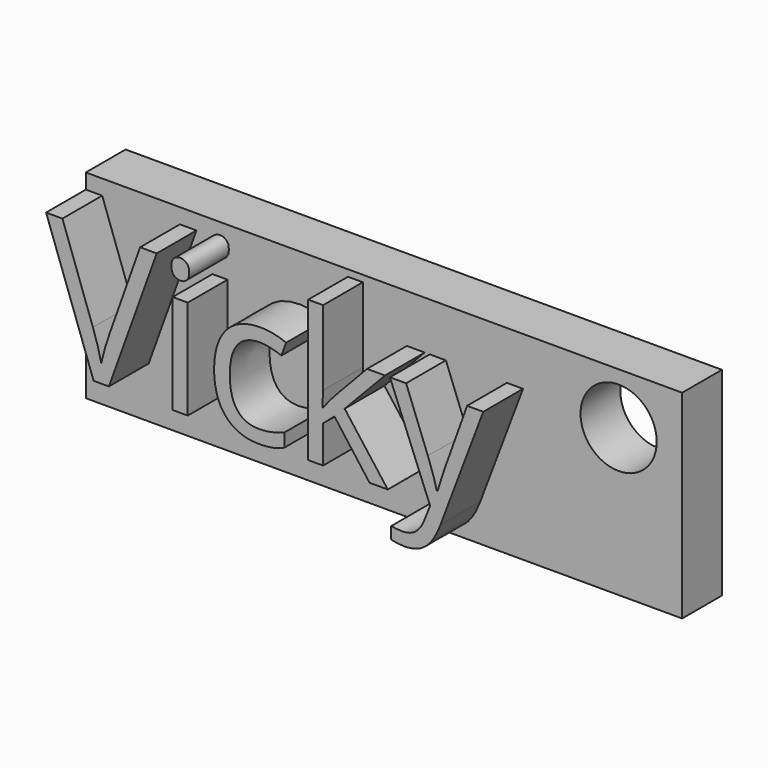
from build123d import *

# Parameters (mm, degrees)
F1_TEXT_SIZE = 23.7509700844
F2_DEPTH     = 12.7
F0_W         = 76.2
F0_H         = 25.4
F3_DEPTH     = 6.35
F4_R         = 4.870183606
F5_DEPTH     = 6.35


# Not quite as in the source:
# - Text() gives the source's letters only with a copy of the font that has no kerning and outlines rounded to 1/6400 em; it was checked with that copy


with BuildPart() as f2:
    # F1 (on face) → F2 (new body)
    with BuildSketch(Plane.XZ):
        with Locations((0, 6.5138929126)):
            Text('Vicky', F1_TEXT_SIZE, font='Open Sans', text_align=(TextAlign.LEFT, TextAlign.BOTTOM))
    extrude(amount=F2_DEPTH)


with BuildPart() as f3:
    # F0 (on Front) → F3 (new body)
    with BuildSketch(Plane.XZ):
        with Locations((38.1, 12.7)):
            Rectangle(F0_W, F0_H)
    extrude(amount=F3_DEPTH)

    # F4 (on face) → F5 (cut, through all)
    with BuildSketch(Plane.XZ.offset(6.35)):
        with Locations((68.0822506547, 18.8198536634)):
            Circle(F4_R)
    extrude(amount=-F5_DEPTH, mode=Mode.SUBTRACT)


solid = Compound([f2.part, f3.part])
